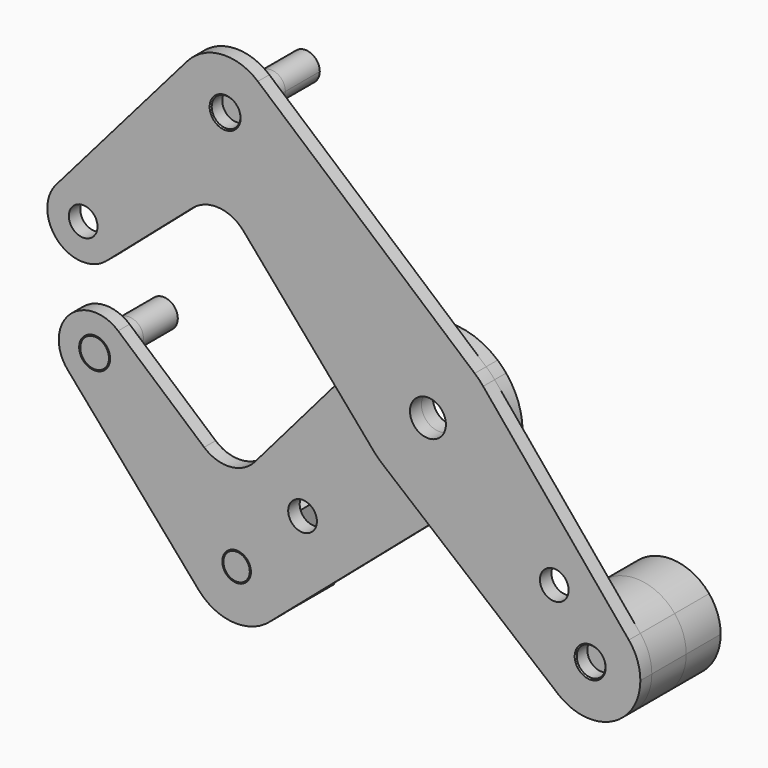
from build123d import *

# Parameters (mm, degrees)
F0_R            = 3.175
F1_DEPTH        = 3.175
F2_DEPTH        = 3.175
F4_DEPTH        = 9.525
F4_COPIES_COUNT = 2
F4_COPIES_PITCH = 9.525
F6_SIZE         = 0.254
F6_2_SIZE       = 0.254
F6_3_SIZE       = 0.254


# Not quite as in the source:
# - a pattern or mirror of a feature is missing from the dataset's text; its kind, count and spacing are read off the source's solid


with BuildPart() as f1:
    # F0 (on Front) → F1 (new body)
    with BuildSketch(Plane.XZ):
        with BuildLine():
            ThreePointArc((-12.0356034274, 10.3518054047), (-11.6386596495, 10.7961672163), (-11.2253201513, 11.2253201513))
            Line((-11.2253201513, 11.2253201513), (-37.0435564994, 37.0435564994))
            ThreePointArc((-37.0435564994, 37.0435564994), (-52.4731730166, 36.7677634349), (-53.300199871, 52.1776678558))
            Line((-53.300199871, 52.1776678558), (-82.331405076, 18.6678036462))
            ThreePointArc((-82.331405076, 18.6678036462), (-73.5586383483, 20.9075469092), (-68.3946770291, 13.4703841816))
            ThreePointArc((-68.3946770291, 13.4703841816), (-69.1121208226, 10.1727039932), (-71.1347575644, 7.4711561347))
            Line((-71.1347575644, 7.4711561347), (-52.0843267669, 23.9754595323))
            ThreePointArc((-52.0843267669, 23.9754595323), (-46.2965222838, 25.8954961667), (-40.8511612346, 23.1508168672))
            Line((-40.8511612346, 23.1508168672), (-20.9391765456, 0))
            Line((-20.9391765456, 0), (-12.0356034274, 10.3518054047))
        make_face()
        with BuildLine():
            ThreePointArc((-53.300199871, 52.1776678558), (-52.4731730166, 36.7677634349), (-37.0435564994, 37.0435564994))
            ThreePointArc((-37.0435564994, 37.0435564994), (-34.6346693003, 40.6487109632), (-33.7887806053, 44.9012806053))
            ThreePointArc((-33.7887806053, 44.9012806053), (-34.8014845049, 49.5361241819), (-37.655016822, 53.3262030046))
            ThreePointArc((-37.655016822, 53.3262030046), (-45.7148756595, 55.9839571475), (-53.300199871, 52.1776678558))
        make_face()
        with BuildLine():
            ThreePointArc((-41.7262806053, 44.9012806053), (-41.9679630896, 43.6862607076), (-42.6562165751, 42.6562165751))
            ThreePointArc((-42.6562165751, 42.6562165751), (-47.8345981211, 46.1163005031), (-41.7262806053, 44.9012806053))
        make_face(mode=Mode.SUBTRACT)
        with BuildLine():
            ThreePointArc((-68.3946770291, 13.4703841816), (-73.5586383483, 20.9075469092), (-82.331405076, 18.6678036462))
            ThreePointArc((-82.331405076, 18.6678036462), (-81.9448371048, 7.8577241059), (-71.1347575644, 7.4711561347))
            ThreePointArc((-71.1347575644, 7.4711561347), (-69.1121208226, 10.1727039932), (-68.3946770291, 13.4703841816))
        make_face()
        with Locations((-76.3321770291, 13.4703841816)):
            Circle(F0_R, mode=Mode.SUBTRACT)
        with BuildLine():
            Line((-37.0435564994, 37.0435564994), (-11.2253201513, 11.2253201513))
            ThreePointArc((-11.2253201513, 11.2253201513), (-0.5957321126, 15.8638182116), (10.3518054047, 12.0356034274))
            Line((10.3518054047, 12.0356034274), (-37.655016822, 53.3262030046))
            ThreePointArc((-37.655016822, 53.3262030046), (-34.8014845049, 49.5361241819), (-33.7887806053, 44.9012806053))
            ThreePointArc((-33.7887806053, 44.9012806053), (-34.6346693003, 40.6487109632), (-37.0435564994, 37.0435564994))
        make_face()
        with BuildLine():
            ThreePointArc((10.3518054047, 12.0356034274), (-0.5957321126, 15.8638182116), (-11.2253201513, 11.2253201513))
            ThreePointArc((-11.2253201513, 11.2253201513), (-11.6386596495, 10.7961672163), (-12.0356034274, 10.3518054047))
            ThreePointArc((-12.0356034274, 10.3518054047), (-15.875, 0), (-12.0356034274, -10.3518054047))
            ThreePointArc((-12.0356034274, -10.3518054047), (-11.1192092809, -11.3304373246), (-10.1235074968, -12.2282550252))
            ThreePointArc((-10.1235074968, -12.2282550252), (0.1493607821, -15.87429735), (10.3518054047, -12.0356034274))
            ThreePointArc((10.3518054047, -12.0356034274), (14.4282801435, -6.6212051093), (15.875, 0))
            ThreePointArc((15.875, 0), (14.9355142785, 5.3801522504), (12.2282550252, 10.1235074968))
            ThreePointArc((12.2282550252, 10.1235074968), (11.3304373246, 11.1192092809), (10.3518054047, 12.0356034274))
        make_face()
        with BuildLine():
            ThreePointArc((3.9751, 0), (-1.521204912, -3.6725135297), (-2.8108201659, 2.8108201659))
            ThreePointArc((-2.8108201659, 2.8108201659), (1.521204912, 3.6725135297), (3.9751, 0))
        make_face(mode=Mode.SUBTRACT)
        with BuildLine():
            ThreePointArc((10.3518054047, -12.0356034274), (0.1493607821, -15.87429735), (-10.1235074968, -12.2282550252))
            Line((-10.1235074968, -12.2282550252), (0.1954344954, -20.7710836138))
            Line((0.1954344954, -20.7710836138), (10.3518054047, -12.0356034274))
        make_face()
        with BuildLine():
            ThreePointArc((-12.0356034274, -10.3518054047), (-15.875, 0), (-12.0356034274, 10.3518054047))
            Line((-12.0356034274, 10.3518054047), (-20.9391765456, 0))
            Line((-20.9391765456, 0), (-12.0356034274, -10.3518054047))
        make_face()
        with BuildLine():
            Line((44.4808030019, -28.8345692365), (12.2282550252, 10.1235074968))
            ThreePointArc((12.2282550252, 10.1235074968), (14.9355142785, 5.3801522504), (15.875, 0))
            ThreePointArc((15.875, 0), (14.4282801435, -6.6212051093), (10.3518054047, -12.0356034274))
            Line((10.3518054047, -12.0356034274), (0.1954344954, -20.7710836138))
            Line((0.1954344954, -20.7710836138), (28.8345692365, -44.4808030019))
            ThreePointArc((28.8345692365, -44.4808030019), (28.0633003783, -28.0633003783), (44.4808030019, -28.8345692365))
        make_face()
        with Locations((27.9745180668, -23.4843900063)):
            Circle(F0_R, mode=Mode.SUBTRACT)
        with BuildLine():
            ThreePointArc((47.0335244843, -35.9210244843), (46.3758844792, -32.154917909), (44.4808030019, -28.8345692365))
            ThreePointArc((44.4808030019, -28.8345692365), (28.0633003783, -28.0633003783), (28.8345692365, -44.4808030019))
            ThreePointArc((28.8345692365, -44.4808030019), (40.650687385, -45.9767663811), (47.0335244843, -35.9210244843))
        make_face()
        with Locations((35.9210244843, -35.9210244843)):
            Circle(F0_R, mode=Mode.SUBTRACT)
    extrude(amount=F1_DEPTH)


with BuildPart() as f2:
    # F0 (on Front) → F2 (new body)
    with BuildSketch(Plane.XZ):
        with BuildLine():
            ThreePointArc((-68.3946770291, -13.4703841816), (-69.1121208226, -10.1727039932), (-71.1347575644, -7.4711561347))
            ThreePointArc((-71.1347575644, -7.4711561347), (-81.9448371048, -7.8577241059), (-82.331405076, -18.6678036462))
            ThreePointArc((-82.331405076, -18.6678036462), (-73.5586383483, -20.9075469092), (-68.3946770291, -13.4703841816))
        make_face()
        with Locations((-76.3321770291, -13.4703841816)):
            Circle(F0_R, mode=Mode.SUBTRACT)
        with BuildLine():
            ThreePointArc((-10.1235074968, -12.2282550252), (-11.1192092809, -11.3304373246), (-12.0356034274, -10.3518054047))
            Line((-12.0356034274, -10.3518054047), (-20.9391765456, 0))
            Line((-20.9391765456, 0), (-40.8511612346, -23.1508168672))
            ThreePointArc((-40.8511612346, -23.1508168672), (-46.2965222838, -25.8954961667), (-52.0843267669, -23.9754595323))
            Line((-52.0843267669, -23.9754595323), (-71.1347575644, -7.4711561347))
            ThreePointArc((-71.1347575644, -7.4711561347), (-69.1121208226, -10.1727039932), (-68.3946770291, -13.4703841816))
            ThreePointArc((-68.3946770291, -13.4703841816), (-73.5586383483, -20.9075469092), (-82.331405076, -18.6678036462))
            Line((-82.331405076, -18.6678036462), (-53.300199871, -52.1776678558))
            ThreePointArc((-53.300199871, -52.1776678558), (-53.1629839096, -37.469462876), (-38.5512806053, -35.781787404))
            ThreePointArc((-38.5512806053, -35.781787404), (-35.0511021488, -39.757192676), (-33.7887806053, -44.9012806053))
            ThreePointArc((-33.7887806053, -44.9012806053), (-34.8014845049, -49.5361241819), (-37.655016822, -53.3262030046))
            Line((-37.655016822, -53.3262030046), (0.1954344954, -20.7710836138))
            Line((0.1954344954, -20.7710836138), (-10.1235074968, -12.2282550252))
        make_face()
        with Locations((-30.2993841525, -30.2993841525)):
            Circle(F0_R, mode=Mode.SUBTRACT)
        with BuildLine():
            ThreePointArc((-53.300199871, -52.1776678558), (-46.2792419349, -55.9280153362), (-38.5512806053, -54.0207738067))
            Line((-38.5512806053, -54.0207738067), (-38.5512806053, -35.781787404))
            ThreePointArc((-38.5512806053, -35.781787404), (-53.1629839096, -37.469462876), (-53.300199871, -52.1776678558))
        make_face()
        with Locations((-44.9012806053, -44.9012806053)):
            Circle(F0_R, mode=Mode.SUBTRACT)
        with BuildLine():
            ThreePointArc((10.3518054047, 12.0356034274), (-0.5957321126, 15.8638182116), (-11.2253201513, 11.2253201513))
            ThreePointArc((-11.2253201513, 11.2253201513), (-11.6386596495, 10.7961672163), (-12.0356034274, 10.3518054047))
            ThreePointArc((-12.0356034274, 10.3518054047), (-15.875, 0), (-12.0356034274, -10.3518054047))
            ThreePointArc((-12.0356034274, -10.3518054047), (-11.1192092809, -11.3304373246), (-10.1235074968, -12.2282550252))
            ThreePointArc((-10.1235074968, -12.2282550252), (0.1493607821, -15.87429735), (10.3518054047, -12.0356034274))
            ThreePointArc((10.3518054047, -12.0356034274), (14.4282801435, -6.6212051093), (15.875, 0))
            ThreePointArc((15.875, 0), (14.9355142785, 5.3801522504), (12.2282550252, 10.1235074968))
            ThreePointArc((12.2282550252, 10.1235074968), (11.3304373246, 11.1192092809), (10.3518054047, 12.0356034274))
        make_face()
        with BuildLine():
            ThreePointArc((3.9751, 0), (-1.521204912, -3.6725135297), (-2.8108201659, 2.8108201659))
            ThreePointArc((-2.8108201659, 2.8108201659), (1.521204912, 3.6725135297), (3.9751, 0))
        make_face(mode=Mode.SUBTRACT)
        with BuildLine():
            ThreePointArc((10.3518054047, -12.0356034274), (0.1493607821, -15.87429735), (-10.1235074968, -12.2282550252))
            Line((-10.1235074968, -12.2282550252), (0.1954344954, -20.7710836138))
            Line((0.1954344954, -20.7710836138), (10.3518054047, -12.0356034274))
        make_face()
        with BuildLine():
            ThreePointArc((-12.0356034274, -10.3518054047), (-15.875, 0), (-12.0356034274, 10.3518054047))
            Line((-12.0356034274, 10.3518054047), (-20.9391765456, 0))
            Line((-20.9391765456, 0), (-12.0356034274, -10.3518054047))
        make_face()
        with BuildLine():
            ThreePointArc((-38.5512806053, -54.0207738067), (-38.0942838839, -53.6849274496), (-37.655016822, -53.3262030046))
            ThreePointArc((-37.655016822, -53.3262030046), (-34.8014845049, -49.5361241819), (-33.7887806053, -44.9012806053))
            ThreePointArc((-33.7887806053, -44.9012806053), (-35.0511021488, -39.757192676), (-38.5512806053, -35.781787404))
            Line((-38.5512806053, -35.781787404), (-38.5512806053, -54.0207738067))
        make_face()
    extrude(amount=-F2_DEPTH)


with BuildPart() as f4:
    # F0 (on Front) → F4 (new body, through all)
    with BuildSketch(Plane.XZ):
        with BuildLine():
            ThreePointArc((-53.300199871, -52.1776678558), (-46.2792419349, -55.9280153362), (-38.5512806053, -54.0207738067))
            Line((-38.5512806053, -54.0207738067), (-38.5512806053, -35.781787404))
            ThreePointArc((-38.5512806053, -35.781787404), (-53.1629839096, -37.469462876), (-53.300199871, -52.1776678558))
        make_face()
        with Locations((-44.9012806053, -44.9012806053)):
            Circle(F0_R, mode=Mode.SUBTRACT)
        with Locations((-44.9012806053, -44.9012806053)):
            Circle(F0_R)
    extrude(amount=-F4_DEPTH)


with BuildPart() as f4b:
    # F0 (on Front) → F4, piece 2 (new body, through all)
    with BuildSketch(Plane.XZ):
        with BuildLine():
            ThreePointArc((47.0335244843, -35.9210244843), (46.3758844792, -32.154917909), (44.4808030019, -28.8345692365))
            ThreePointArc((44.4808030019, -28.8345692365), (28.0633003783, -28.0633003783), (28.8345692365, -44.4808030019))
            ThreePointArc((28.8345692365, -44.4808030019), (40.650687385, -45.9767663811), (47.0335244843, -35.9210244843))
        make_face()
        with Locations((35.9210244843, -35.9210244843)):
            Circle(F0_R, mode=Mode.SUBTRACT)
        with Locations((35.9210244843, -35.9210244843)):
            Circle(F0_R)
    extrude(amount=-F4_DEPTH)


with BuildPart() as f4c:
    # F0 (on Front) → F4, piece 3 (new body, through all)
    with BuildSketch(Plane.XZ):
        with BuildLine():
            ThreePointArc((-41.7262806053, 44.9012806053), (-47.8345981211, 46.1163005031), (-42.6562165751, 42.6562165751))
            ThreePointArc((-42.6562165751, 42.6562165751), (-41.9679630896, 43.6862607076), (-41.7262806053, 44.9012806053))
        make_face()
    extrude(amount=-F4_DEPTH)


with BuildPart() as f4d:
    # F0 (on Front) → F4, piece 4 (new body, through all)
    with BuildSketch(Plane.XZ):
        with Locations((-76.3321770291, -13.4703841816)):
            Circle(F0_R)
    extrude(amount=-F4_DEPTH)


with BuildPart() as f4_copies_1:
    # F4_copies: instance of F4
    add(f4.part.moved(Location(Vector(0, 1, 0) * (1 * F4_COPIES_PITCH))))


with BuildPart() as f4_2_copies_1:
    # F4_2_copies: instance of F4b
    add(f4b.part.mirror(Plane.ZX.offset(9.525)))


with BuildPart() as f4_3_copies_1:
    # F4_3_copies: instance of F4c
    add(f4c.part.mirror(Plane.ZX.offset(9.525)))


with BuildPart() as f4_4_copies_1:
    # F4_4_copies: instance of F4d
    add(f4d.part.mirror(Plane.ZX.offset(9.525)))


with BuildPart() as f4c_1:
    add(f4c.part)

    # F5: cut F1, F2
    add(f1.part, mode=Mode.SUBTRACT)
    add(f2.part, mode=Mode.SUBTRACT)


with BuildPart() as f4b_1:
    add(f4b.part)

    # F5: cut F1, F2
    add(f1.part, mode=Mode.SUBTRACT)
    add(f2.part, mode=Mode.SUBTRACT)


with BuildPart() as f4_1:
    add(f4.part)

    # F5: cut F1, F2
    add(f1.part, mode=Mode.SUBTRACT)
    add(f2.part, mode=Mode.SUBTRACT)

    # F6#3
    f6_3_edges = [f4_1.edges().sort_by_distance(p)[0] for p in [
        (-48.076281, 0, -44.901281),
    ]]
    chamfer(f6_3_edges, length=F6_3_SIZE)


with BuildPart() as f4d_1:
    add(f4d.part)

    # F5: cut F1, F2
    add(f1.part, mode=Mode.SUBTRACT)
    add(f2.part, mode=Mode.SUBTRACT)


with BuildPart() as f1_1:
    add(f1.part)

    # F6
    f6_edges = [f1_1.edges().sort_by_distance(p)[0] for p in [
        (-48.076281, -3.175, 44.901281),
        (32.746024, -3.175, -35.921024),
    ]]
    chamfer(f6_edges, length=F6_SIZE)


with BuildPart() as f2_1:
    add(f2.part)

    # F6#2
    f6_2_edges = [f2_1.edges().sort_by_distance(p)[0] for p in [
        (-79.507177, 0, -13.470384),
    ]]
    chamfer(f6_2_edges, length=F6_2_SIZE)


solid = Compound([f4_copies_1.part, f4_2_copies_1.part, f4_3_copies_1.part, f4_4_copies_1.part, f4c_1.part, f4b_1.part, f4_1.part, f4d_1.part, f1_1.part, f2_1.part])
